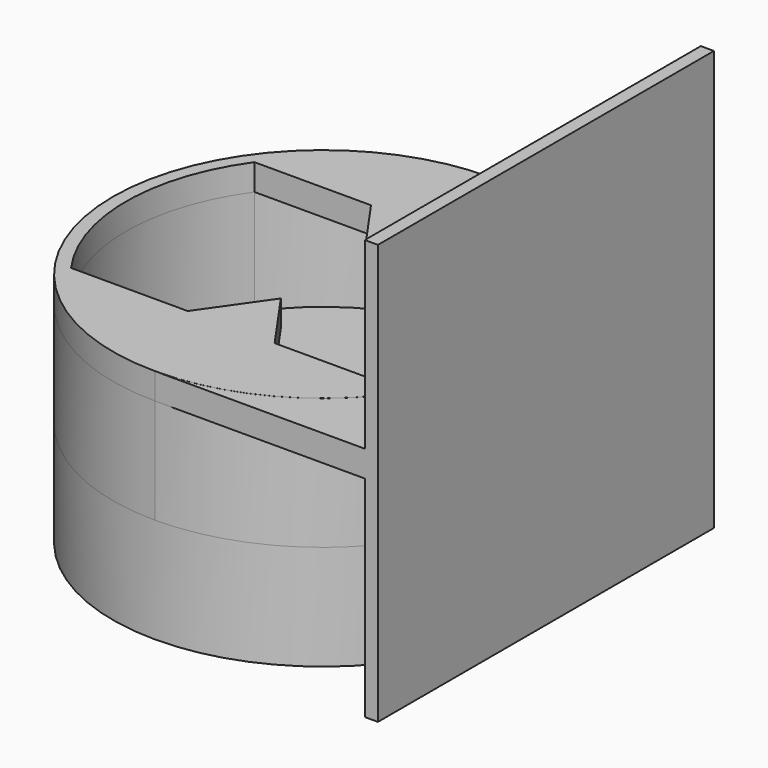
from build123d import *
from build123d import SkipClean  # not in build123d's __all__

# Parameters (mm, degrees)
F1_DEPTH = 50.8
F2_DEPTH = 6.35
F3_DEPTH = 25.4
F4_R     = 50.7746
F4_R_2   = 47.625
F4_R_3   = 12.7
F5_DEPTH = 25.4


# Not quite as in the source:
# - after a boolean that leaves OpenCascade's solid faulty, fix() repairs it


with BuildPart() as f1:
    # F0 (on Top) → F1 (new body, symmetric)
    with BuildSketch(Plane.XY):
        Polygon((50.8, 50.8), (50.8, 0), (50.8, -50.8), (53.975, -50.8), (53.975, 50.8), align=None)
    extrude(amount=F1_DEPTH, both=True)

    # F0 (on Top) → F2 (join)
    with BuildSketch(Plane.XY):
        with BuildLine():
            Line((50.8, 50.8), (0, 50.8))
            ThreePointArc((0, 50.8), (35.9210244843, 35.9210244843), (50.8, 0))
            Line((50.8, 0), (50.8, 50.8))
        make_face()
        with BuildLine():
            ThreePointArc((50.8, 0), (35.9210244843, -35.9210244843), (0, -50.8))
            Line((0, -50.8), (50.8, -50.8))
            Line((50.8, -50.8), (50.8, 0))
        make_face()
    extrude(amount=F2_DEPTH)


with BuildPart() as f2:
    # F0 (on Top) → F2, piece 2 (new body)
    with BuildSketch(Plane.XY):
        with BuildLine():
            ThreePointArc((38.7296379439, 27.7156232067), (45.3466626781, 14.5540650322), (47.625, 0))
            ThreePointArc((47.625, 0), (45.3466626781, -14.5540650322), (38.7296379439, -27.7156232067))
            ThreePointArc((38.7296379439, -27.7156232067), (30.8076970757, -36.318403405), (21.0281051205, -42.7312464134))
            ThreePointArc((21.0281051205, -42.7312464134), (10.7950223382, -46.3854300155), (0, -47.625))
            Line((0, -47.625), (0, -50.7746))
            ThreePointArc((0, -50.7746), (35.903063972, -35.903063972), (50.7746, 0))
            ThreePointArc((50.7746, 0), (35.903063972, 35.903063972), (0, 50.7746))
            Line((0, 50.7746), (0, 47.625))
            ThreePointArc((0, 47.625), (10.7950223382, 46.3854300155), (21.0281051205, 42.7312464134))
            ThreePointArc((21.0281051205, 42.7312464134), (30.8076970757, 36.318403405), (38.7296379439, 27.7156232067))
        make_face()
        with BuildLine():
            ThreePointArc((-21.0281051205, 42.7312464134), (-10.7950223382, 46.3854300155), (0, 47.625))
            Line((0, 47.625), (0, 50.7746))
            ThreePointArc((0, 50.7746), (-50.7746, 0), (0, -50.7746))
            Line((0, -50.7746), (0, -47.625))
            ThreePointArc((0, -47.625), (-10.7950223382, -46.3854300155), (-21.0281051205, -42.7312464134))
            ThreePointArc((-21.0281051205, -42.7312464134), (-30.8076970757, -36.318403405), (-38.7296379439, -27.7156232067))
            ThreePointArc((-38.7296379439, -27.7156232067), (-47.625, 0), (-38.7296379439, 27.7156232067))
            ThreePointArc((-38.7296379439, 27.7156232067), (-30.8076970757, 36.318403405), (-21.0281051205, 42.7312464134))
        make_face()
        with BuildLine():
            Line((-10.5140525602, 27.7156232067), (-21.0281051205, 42.7312464134))
            ThreePointArc((-21.0281051205, 42.7312464134), (-30.8076970757, 36.318403405), (-38.7296379439, 27.7156232067))
            Line((-38.7296379439, 27.7156232067), (-10.5140525602, 27.7156232067))
        make_face()
        with BuildLine():
            Line((0, 12.7), (0, 47.625))
            ThreePointArc((0, 47.625), (-10.7950223382, 46.3854300155), (-21.0281051205, 42.7312464134))
            Line((-21.0281051205, 42.7312464134), (-10.5140525602, 27.7156232067))
            Line((-10.5140525602, 27.7156232067), (0, 12.7))
        make_face()
        with BuildLine():
            Line((10.5140525602, 27.7156232067), (21.0281051205, 42.7312464134))
            ThreePointArc((21.0281051205, 42.7312464134), (10.7950223382, 46.3854300155), (0, 47.625))
            Line((0, 47.625), (0, 12.7))
            Line((0, 12.7), (10.5140525602, 27.7156232067))
        make_face()
        with BuildLine():
            Line((10.5140525602, 27.7156232067), (38.7296379439, 27.7156232067))
            ThreePointArc((38.7296379439, 27.7156232067), (30.8076970757, 36.318403405), (21.0281051205, 42.7312464134))
            Line((21.0281051205, 42.7312464134), (10.5140525602, 27.7156232067))
        make_face()
        with BuildLine():
            ThreePointArc((21.0281051205, -42.7312464134), (30.8076970757, -36.318403405), (38.7296379439, -27.7156232067))
            Line((38.7296379439, -27.7156232067), (10.5140525602, -27.7156232067))
            Line((10.5140525602, -27.7156232067), (21.0281051205, -42.7312464134))
        make_face()
        with BuildLine():
            ThreePointArc((0, -47.625), (10.7950223382, -46.3854300155), (21.0281051205, -42.7312464134))
            Line((21.0281051205, -42.7312464134), (10.5140525602, -27.7156232067))
            Line((10.5140525602, -27.7156232067), (0, -12.7))
            Line((0, -12.7), (0, -47.625))
        make_face()
        with BuildLine():
            ThreePointArc((-21.0281051205, -42.7312464134), (-10.7950223382, -46.3854300155), (0, -47.625))
            Line((0, -47.625), (0, -12.7))
            Line((0, -12.7), (-10.5140525602, -27.7156232067))
            Line((-10.5140525602, -27.7156232067), (-21.0281051205, -42.7312464134))
        make_face()
        with BuildLine():
            ThreePointArc((-38.7296379439, -27.7156232067), (-30.8076970757, -36.318403405), (-21.0281051205, -42.7312464134))
            Line((-21.0281051205, -42.7312464134), (-10.5140525602, -27.7156232067))
            Line((-10.5140525602, -27.7156232067), (-38.7296379439, -27.7156232067))
        make_face()
    extrude(amount=F2_DEPTH)

    # F0 (on Top) → F3 (join)
    with BuildSketch(Plane.XY):
        with BuildLine():
            ThreePointArc((-21.0281051205, 42.7312464134), (-10.7950223382, 46.3854300155), (0, 47.625))
            Line((0, 47.625), (0, 50.7746))
            ThreePointArc((0, 50.7746), (-50.7746, 0), (0, -50.7746))
            Line((0, -50.7746), (0, -47.625))
            ThreePointArc((0, -47.625), (-10.7950223382, -46.3854300155), (-21.0281051205, -42.7312464134))
            ThreePointArc((-21.0281051205, -42.7312464134), (-30.8076970757, -36.318403405), (-38.7296379439, -27.7156232067))
            ThreePointArc((-38.7296379439, -27.7156232067), (-47.625, 0), (-38.7296379439, 27.7156232067))
            ThreePointArc((-38.7296379439, 27.7156232067), (-30.8076970757, 36.318403405), (-21.0281051205, 42.7312464134))
        make_face()
        with BuildLine():
            ThreePointArc((38.7296379439, 27.7156232067), (45.3466626781, 14.5540650322), (47.625, 0))
            ThreePointArc((47.625, 0), (45.3466626781, -14.5540650322), (38.7296379439, -27.7156232067))
            ThreePointArc((38.7296379439, -27.7156232067), (30.8076970757, -36.318403405), (21.0281051205, -42.7312464134))
            ThreePointArc((21.0281051205, -42.7312464134), (10.7950223382, -46.3854300155), (0, -47.625))
            Line((0, -47.625), (0, -50.7746))
            ThreePointArc((0, -50.7746), (35.903063972, -35.903063972), (50.7746, 0))
            ThreePointArc((50.7746, 0), (35.903063972, 35.903063972), (0, 50.7746))
            Line((0, 50.7746), (0, 47.625))
            ThreePointArc((0, 47.625), (10.7950223382, 46.3854300155), (21.0281051205, 42.7312464134))
            ThreePointArc((21.0281051205, 42.7312464134), (30.8076970757, 36.318403405), (38.7296379439, 27.7156232067))
        make_face()
    with SkipClean():  # cleaning this boolean's faces spoils the solid; the shape is the same uncleaned
        extrude(amount=-F3_DEPTH)

    # F4 (on face) → F5 (join)
    with BuildSketch(Plane(origin=(0, 0, -25.4), x_dir=(1, 0, 0), z_dir=(0, 0, -1))):
        Circle(F4_R)
        Circle(F4_R_2, mode=Mode.SUBTRACT)
        Circle(F4_R_2)
        Circle(F4_R_3, mode=Mode.SUBTRACT)
    extrude(amount=F5_DEPTH)

    add(f2.part.fix(), mode=Mode.REPLACE)


solid = Compound([f1.part, f2.part])
